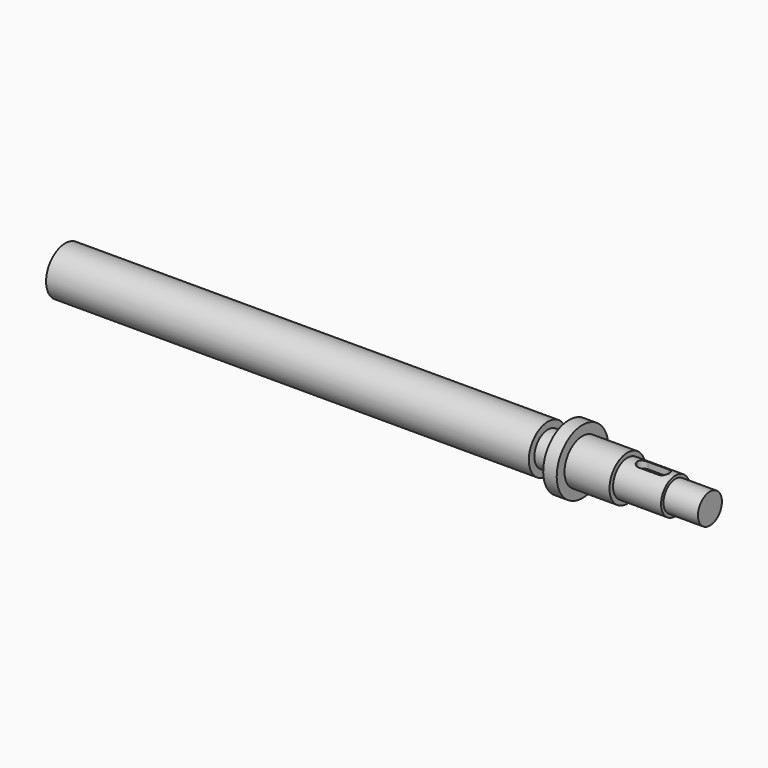
from build123d import *

# Parameters (mm, degrees)
F3_W     = 10.7
F3_H     = 4
F4_DEPTH = 4
F5_R     = 1.99999


# Not quite as in the source:
# - a fillet or chamfer is up to 0.001 mm smaller than in the source, because OpenCascade refuses the exact size


with BuildPart() as f1:
    # F0 (on Front) → F1 (revolve)
    with BuildSketch(Plane.XZ):
        Polygon((0, 8), (0, 0), (215, 0), (215, 5), (203.5, 5), (203.5, 6), (187.5, 6), (187.5, 7.5), (172.5, 7.5), (172.5, 10.75), (168, 10.75), (168, 5.675), (161, 5.675), (161, 8), align=None)
    revolve(axis=Axis((-30.1147408886, 0, 0), (-1, 0, 0)))

    # F3 (on offset) → F4 (cut)
    with BuildSketch(Plane.XY.offset(7.5)):
        with Locations((196.15, 0)):
            Rectangle(F3_W, F3_H)
    extrude(amount=-F4_DEPTH, mode=Mode.SUBTRACT)

    # F5 (radius 2 in the source; OpenCascade refuses exactly that, so slightly less here)
    f5_edges = [f1.edges().sort_by_distance(p)[0] for p in [
        (190.8, 2, 4.578427),
        (201.5, 2, 4.578427),
        (201.5, -2, 4.578427),
        (190.8, -2, 4.578427),
    ]]
    fillet(f5_edges, radius=F5_R)


solid = f1.part
